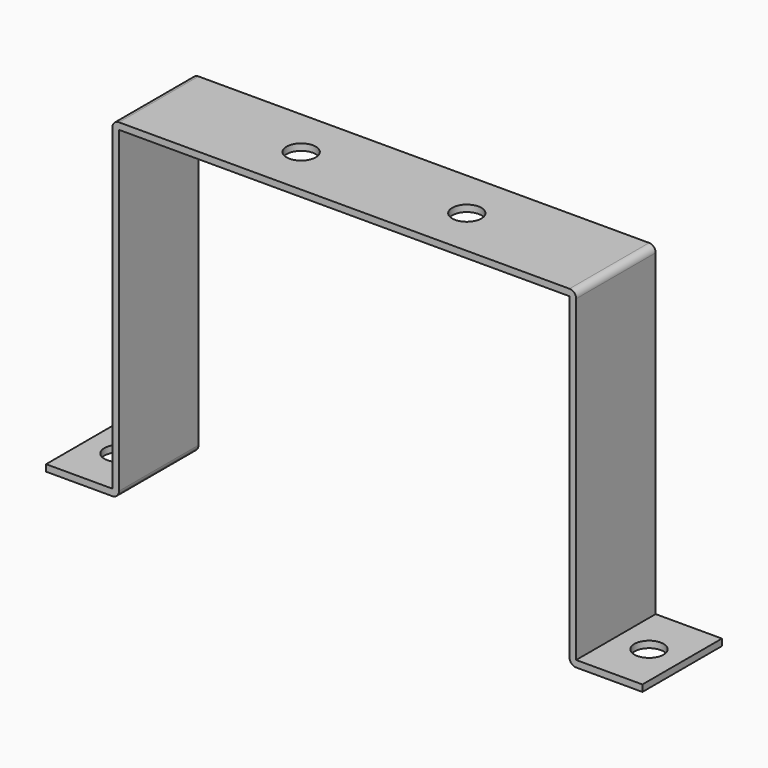
from build123d import *

# Parameters (mm, degrees)
F1_DEPTH = 30
F2_R     = 4.4
F3_R     = 4.4
F4_DEPTH = 25
F5_R     = 2
F6_R     = 2


# Not quite as in the source:
# - a feature names something its author has since deleted; it is built from what else it names


with BuildPart() as f1:
    # F0 (on Front) → F1 (new body)
    with BuildSketch(Plane.XZ):
        Polygon((90, -1), (90, 1), (70, 1), (70, 99), (-70, 99), (-70, 1), (-90, 1), (-90, -1), (-68, -1), (-68, 97), (68, 97), (68, -1), align=None)
    extrude(amount=F1_DEPTH)

    # F2 (on face) + F3 (on face) → F4 (cut)
    with BuildSketch(Plane.XY.offset(1)):
        with Locations((-80, -15)):
            Circle(F2_R)
        with Locations((80, -15)):
            Circle(F2_R)
    with BuildSketch(Plane.XY.offset(99)):
        with Locations((-25, -15)):
            Circle(F3_R)
        with Locations((25, -15)):
            Circle(F3_R)
    extrude(amount=-F4_DEPTH, mode=Mode.SUBTRACT)

    # F5
    f5_edges = [f1.edges().sort_by_distance(p)[0] for p in [
        (-70, -15, 99),
        (70, -15, 99),
    ]]
    fillet(f5_edges, radius=F5_R)

    # F6
    f6_edges = [f1.edges().sort_by_distance(p)[0] for p in [
        (68, -15, -1),
        (-68, -15, -1),
    ]]
    fillet(f6_edges, radius=F6_R)


solid = f1.part
